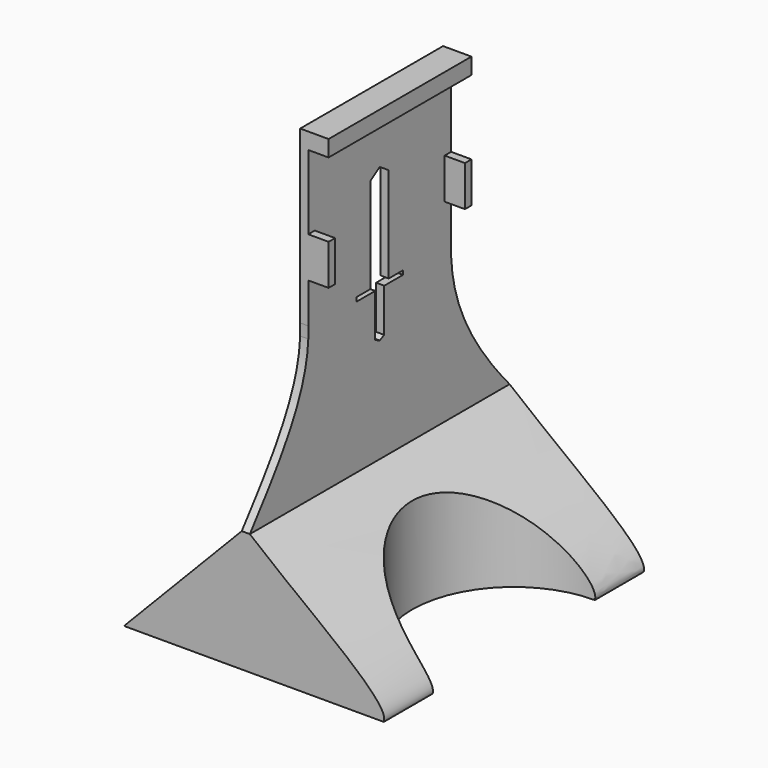
from build123d import *

# Parameters (mm, degrees)
F1_DEPTH  = 400
F2_R      = 75
F2_R_2    = 125
F3_DEPTH  = 160
F4_W      = 10
F4_H      = 400
F5_DEPTH  = 400
F7_DEPTH  = 369
F8_DEPTH  = 744
F9_DEPTH  = 294
F10_DEPTH = 25
F11_W     = 220
F11_H     = 20
F12_DEPTH = 25
F13_W     = 10
F13_H     = 50
F14_DEPTH = 25


with BuildPart() as f1:
    # F0 (on Front) → F1 (new body)
    with BuildSketch(Plane.XZ):
        with BuildLine():
            Line((-10, 0), (0, 0))
            Line((0, 0), (160, 0))
            add(Edge.make_bspline(
                [(160, 0), (168.8577404315, 22.9710926099), (70.8040622396, 86.9003880522), (-4.9911788106, 150)],
                knots=[0.4586039165, 0.4586039165, 0.4586039165, 0.4586039165, 1, 1, 1, 1], degree=3))
            Line((-4.9911788106, 150), (-14.9911788106, 150))
            Line((-14.9911788106, 150), (-160, 0))
            Line((-160, 0), (-60, 0))
            Line((-60, 0), (-10, 0))
        make_face()
    extrude(amount=F1_DEPTH)

    # F2 (on face) → F3 (cut)
    with BuildSketch(Plane(origin=(0, 0, 0), x_dir=(1, 0, 0), z_dir=(0, 0, -1))):
        with Locations((-160, 200)):
            Circle(F2_R)
        with Locations((160, 200)):
            Circle(F2_R_2)
    extrude(amount=-F3_DEPTH, mode=Mode.SUBTRACT)

    # F4 (on face) → F5 (join)
    with BuildSketch(Plane.XY.offset(150)):
        with Locations((-9.9911788106, -200)):
            Rectangle(F4_W, F4_H)
    extrude(amount=F5_DEPTH)

    # F6 (on face) → F7 (cut)
    with BuildSketch(Plane.YZ.offset(-4.9911788106)):
        with BuildLine():
            Line((-400, 550), (-400, 150))
            add(Edge.make_bspline(
                [(-400, 150), (-356.3451728041, 206.1467944777), (-312.9584078924, 262.3039541318), (-310, 325.0278234482)],
                knots=[0, 0, 0, 0, 0.4740286783, 0.4740286783, 0.4740286783, 0.4740286783], degree=3))
            Line((-310, 325.0278234482), (-310, 339.2202581751))
            add(Edge.make_bspline(
                [(-310, 339.2202581751), (-312.9911644459, 405.1052836748), (-356.3650932552, 477.5474537124), (-400, 550)],
                knots=[0.5095094707, 0.5095094707, 0.5095094707, 0.5095094707, 1, 1, 1, 1], degree=3))
        make_face()
        with BuildLine():
            Line((0, 550), (-90, 550))
            Line((-90, 550), (-90, 530))
            Line((-90, 530), (-90, 340.4403127563))
            add(Edge.make_bspline(
                [(0, 550), (-49.5785227153, 477.7428221558), (-87.2010209493, 405.969304948), (-90, 340.4403127563)],
                knots=[0, 0, 0, 0, 0.4874574601, 0.4874574601, 0.4874574601, 0.4874574601], degree=3))
        make_face()
        with BuildLine():
            Line((-310, 339.2202581751), (-310, 325.0278234482))
            add(Edge.make_bspline(
                [(-310, 325.0278234482), (-309.7785647553, 329.7226714383), (-309.7836270458, 334.4543090401), (-310, 339.2202581751)],
                knots=[0.4740286783, 0.4740286783, 0.4740286783, 0.4740286783, 0.5095094707, 0.5095094707, 0.5095094707, 0.5095094707], degree=3))
        make_face()
        with BuildLine():
            Line((-310, 550), (-400, 550))
            add(Edge.make_bspline(
                [(-310, 339.2202581751), (-312.9911644459, 405.1052836748), (-356.3650932552, 477.5474537124), (-400, 550)],
                knots=[0.5095094707, 0.5095094707, 0.5095094707, 0.5095094707, 1, 1, 1, 1], degree=3))
            Line((-310, 339.2202581751), (-310, 530))
            Line((-310, 530), (-310, 550))
        make_face()
        with BuildLine():
            Line((0, 150), (0, 550))
            add(Edge.make_bspline(
                [(0, 550), (-49.5785227153, 477.7428221558), (-87.2010209493, 405.969304948), (-90, 340.4403127563)],
                knots=[0, 0, 0, 0, 0.4874574601, 0.4874574601, 0.4874574601, 0.4874574601], degree=3))
            Line((-90, 340.4403127563), (-90, 325.0278234482))
            add(Edge.make_bspline(
                [(-90, 325.0278234482), (-87.2318561535, 262.2986085933), (-49.8238669759, 205.9050330021), (0, 150)],
                knots=[0.5259713217, 0.5259713217, 0.5259713217, 0.5259713217, 1, 1, 1, 1], degree=3))
        make_face()
        with BuildLine():
            Line((-90, 325.0278234482), (-90, 340.4403127563))
            add(Edge.make_bspline(
                [(-90, 340.4403127563), (-90.2211464603, 335.2628875556), (-90.224906032, 330.1244439943), (-90, 325.0278234482)],
                knots=[0.4874574601, 0.4874574601, 0.4874574601, 0.4874574601, 0.5259713217, 0.5259713217, 0.5259713217, 0.5259713217], degree=3))
        make_face()
        Polygon((-186.1447365284, 340.2760970592), (-186.1447365284, 457.7941475637), (-200, 466.9407904148), (-213.8552634716, 457.7941475637), (-213.8552634716, 340.2760970592), (-225.8552634716, 340.2760970592), (-235.8552634716, 340.2760970592), (-235.8552634716, 335.2760970592), (-213.8552634716, 335.2760970592), (-206.9276317358, 335.2760970592), (-206.9276317358, 281.9714009762), (-200, 278.6667048931), (-193.0723682642, 281.9714009762), (-193.0723682642, 335.2760970592), (-186.1447365284, 335.2760970592), (-164.1447365284, 335.2760970592), (-164.1447365284, 340.2760970592), (-174.1447365284, 340.2760970592), align=None)
    extrude(amount=-F7_DEPTH, mode=Mode.SUBTRACT)

    # F6 (on face) → F8 (cut)
    with BuildSketch(Plane.YZ.offset(-4.9911788106)):
        with BuildLine():
            Line((-400, 550), (-400, 150))
            add(Edge.make_bspline(
                [(-400, 150), (-356.3451728041, 206.1467944777), (-312.9584078924, 262.3039541318), (-310, 325.0278234482)],
                knots=[0, 0, 0, 0, 0.4740286783, 0.4740286783, 0.4740286783, 0.4740286783], degree=3))
            Line((-310, 325.0278234482), (-310, 339.2202581751))
            add(Edge.make_bspline(
                [(-310, 339.2202581751), (-312.9911644459, 405.1052836748), (-356.3650932552, 477.5474537124), (-400, 550)],
                knots=[0.5095094707, 0.5095094707, 0.5095094707, 0.5095094707, 1, 1, 1, 1], degree=3))
        make_face()
        with BuildLine():
            Line((0, 550), (-90, 550))
            Line((-90, 550), (-90, 530))
            Line((-90, 530), (-90, 340.4403127563))
            add(Edge.make_bspline(
                [(0, 550), (-49.5785227153, 477.7428221558), (-87.2010209493, 405.969304948), (-90, 340.4403127563)],
                knots=[0, 0, 0, 0, 0.4874574601, 0.4874574601, 0.4874574601, 0.4874574601], degree=3))
        make_face()
        with BuildLine():
            Line((-310, 339.2202581751), (-310, 325.0278234482))
            add(Edge.make_bspline(
                [(-310, 325.0278234482), (-309.7785647553, 329.7226714383), (-309.7836270458, 334.4543090401), (-310, 339.2202581751)],
                knots=[0.4740286783, 0.4740286783, 0.4740286783, 0.4740286783, 0.5095094707, 0.5095094707, 0.5095094707, 0.5095094707], degree=3))
        make_face()
        with BuildLine():
            Line((-310, 550), (-400, 550))
            add(Edge.make_bspline(
                [(-310, 339.2202581751), (-312.9911644459, 405.1052836748), (-356.3650932552, 477.5474537124), (-400, 550)],
                knots=[0.5095094707, 0.5095094707, 0.5095094707, 0.5095094707, 1, 1, 1, 1], degree=3))
            Line((-310, 339.2202581751), (-310, 530))
            Line((-310, 530), (-310, 550))
        make_face()
        with BuildLine():
            Line((0, 150), (0, 550))
            add(Edge.make_bspline(
                [(0, 550), (-49.5785227153, 477.7428221558), (-87.2010209493, 405.969304948), (-90, 340.4403127563)],
                knots=[0, 0, 0, 0, 0.4874574601, 0.4874574601, 0.4874574601, 0.4874574601], degree=3))
            Line((-90, 340.4403127563), (-90, 325.0278234482))
            add(Edge.make_bspline(
                [(-90, 325.0278234482), (-87.2318561535, 262.2986085933), (-49.8238669759, 205.9050330021), (0, 150)],
                knots=[0.5259713217, 0.5259713217, 0.5259713217, 0.5259713217, 1, 1, 1, 1], degree=3))
        make_face()
        with BuildLine():
            Line((-90, 325.0278234482), (-90, 340.4403127563))
            add(Edge.make_bspline(
                [(-90, 340.4403127563), (-90.2211464603, 335.2628875556), (-90.224906032, 330.1244439943), (-90, 325.0278234482)],
                knots=[0.4874574601, 0.4874574601, 0.4874574601, 0.4874574601, 0.5259713217, 0.5259713217, 0.5259713217, 0.5259713217], degree=3))
        make_face()
        Polygon((-186.1447365284, 340.2760970592), (-186.1447365284, 457.7941475637), (-200, 466.9407904148), (-213.8552634716, 457.7941475637), (-213.8552634716, 340.2760970592), (-225.8552634716, 340.2760970592), (-235.8552634716, 340.2760970592), (-235.8552634716, 335.2760970592), (-213.8552634716, 335.2760970592), (-206.9276317358, 335.2760970592), (-206.9276317358, 281.9714009762), (-200, 278.6667048931), (-193.0723682642, 281.9714009762), (-193.0723682642, 335.2760970592), (-186.1447365284, 335.2760970592), (-164.1447365284, 335.2760970592), (-164.1447365284, 340.2760970592), (-174.1447365284, 340.2760970592), align=None)
    extrude(amount=-F8_DEPTH, mode=Mode.SUBTRACT)

    # F6 (on face) → F9 (cut)
    with BuildSketch(Plane.YZ.offset(-4.9911788106)):
        with BuildLine():
            Line((-400, 550), (-400, 150))
            add(Edge.make_bspline(
                [(-400, 150), (-356.3451728041, 206.1467944777), (-312.9584078924, 262.3039541318), (-310, 325.0278234482)],
                knots=[0, 0, 0, 0, 0.4740286783, 0.4740286783, 0.4740286783, 0.4740286783], degree=3))
            Line((-310, 325.0278234482), (-310, 339.2202581751))
            add(Edge.make_bspline(
                [(-310, 339.2202581751), (-312.9911644459, 405.1052836748), (-356.3650932552, 477.5474537124), (-400, 550)],
                knots=[0.5095094707, 0.5095094707, 0.5095094707, 0.5095094707, 1, 1, 1, 1], degree=3))
        make_face()
        with BuildLine():
            Line((0, 550), (-90, 550))
            Line((-90, 550), (-90, 530))
            Line((-90, 530), (-90, 340.4403127563))
            add(Edge.make_bspline(
                [(0, 550), (-49.5785227153, 477.7428221558), (-87.2010209493, 405.969304948), (-90, 340.4403127563)],
                knots=[0, 0, 0, 0, 0.4874574601, 0.4874574601, 0.4874574601, 0.4874574601], degree=3))
        make_face()
        with BuildLine():
            Line((-310, 339.2202581751), (-310, 325.0278234482))
            add(Edge.make_bspline(
                [(-310, 325.0278234482), (-309.7785647553, 329.7226714383), (-309.7836270458, 334.4543090401), (-310, 339.2202581751)],
                knots=[0.4740286783, 0.4740286783, 0.4740286783, 0.4740286783, 0.5095094707, 0.5095094707, 0.5095094707, 0.5095094707], degree=3))
        make_face()
        with BuildLine():
            Line((-310, 550), (-400, 550))
            add(Edge.make_bspline(
                [(-310, 339.2202581751), (-312.9911644459, 405.1052836748), (-356.3650932552, 477.5474537124), (-400, 550)],
                knots=[0.5095094707, 0.5095094707, 0.5095094707, 0.5095094707, 1, 1, 1, 1], degree=3))
            Line((-310, 339.2202581751), (-310, 530))
            Line((-310, 530), (-310, 550))
        make_face()
        with BuildLine():
            Line((0, 150), (0, 550))
            add(Edge.make_bspline(
                [(0, 550), (-49.5785227153, 477.7428221558), (-87.2010209493, 405.969304948), (-90, 340.4403127563)],
                knots=[0, 0, 0, 0, 0.4874574601, 0.4874574601, 0.4874574601, 0.4874574601], degree=3))
            Line((-90, 340.4403127563), (-90, 325.0278234482))
            add(Edge.make_bspline(
                [(-90, 325.0278234482), (-87.2318561535, 262.2986085933), (-49.8238669759, 205.9050330021), (0, 150)],
                knots=[0.5259713217, 0.5259713217, 0.5259713217, 0.5259713217, 1, 1, 1, 1], degree=3))
        make_face()
        with BuildLine():
            Line((-90, 325.0278234482), (-90, 340.4403127563))
            add(Edge.make_bspline(
                [(-90, 340.4403127563), (-90.2211464603, 335.2628875556), (-90.224906032, 330.1244439943), (-90, 325.0278234482)],
                knots=[0.4874574601, 0.4874574601, 0.4874574601, 0.4874574601, 0.5259713217, 0.5259713217, 0.5259713217, 0.5259713217], degree=3))
        make_face()
        Polygon((-186.1447365284, 340.2760970592), (-186.1447365284, 457.7941475637), (-200, 466.9407904148), (-213.8552634716, 457.7941475637), (-213.8552634716, 340.2760970592), (-225.8552634716, 340.2760970592), (-235.8552634716, 340.2760970592), (-235.8552634716, 335.2760970592), (-213.8552634716, 335.2760970592), (-206.9276317358, 335.2760970592), (-206.9276317358, 281.9714009762), (-200, 278.6667048931), (-193.0723682642, 281.9714009762), (-193.0723682642, 335.2760970592), (-186.1447365284, 335.2760970592), (-164.1447365284, 335.2760970592), (-164.1447365284, 340.2760970592), (-174.1447365284, 340.2760970592), align=None)
    extrude(amount=-F9_DEPTH, mode=Mode.SUBTRACT)

    # F6 (on face) → F10 (cut)
    with BuildSketch(Plane.YZ.offset(-4.9911788106)):
        with BuildLine():
            Line((-400, 550), (-400, 150))
            add(Edge.make_bspline(
                [(-400, 150), (-356.3451728041, 206.1467944777), (-312.9584078924, 262.3039541318), (-310, 325.0278234482)],
                knots=[0, 0, 0, 0, 0.4740286783, 0.4740286783, 0.4740286783, 0.4740286783], degree=3))
            Line((-310, 325.0278234482), (-310, 339.2202581751))
            add(Edge.make_bspline(
                [(-310, 339.2202581751), (-312.9911644459, 405.1052836748), (-356.3650932552, 477.5474537124), (-400, 550)],
                knots=[0.5095094707, 0.5095094707, 0.5095094707, 0.5095094707, 1, 1, 1, 1], degree=3))
        make_face()
        with BuildLine():
            Line((0, 550), (-90, 550))
            Line((-90, 550), (-90, 530))
            Line((-90, 530), (-90, 340.4403127563))
            add(Edge.make_bspline(
                [(0, 550), (-49.5785227153, 477.7428221558), (-87.2010209493, 405.969304948), (-90, 340.4403127563)],
                knots=[0, 0, 0, 0, 0.4874574601, 0.4874574601, 0.4874574601, 0.4874574601], degree=3))
        make_face()
        with BuildLine():
            Line((-310, 339.2202581751), (-310, 325.0278234482))
            add(Edge.make_bspline(
                [(-310, 325.0278234482), (-309.7785647553, 329.7226714383), (-309.7836270458, 334.4543090401), (-310, 339.2202581751)],
                knots=[0.4740286783, 0.4740286783, 0.4740286783, 0.4740286783, 0.5095094707, 0.5095094707, 0.5095094707, 0.5095094707], degree=3))
        make_face()
        with BuildLine():
            Line((-310, 550), (-400, 550))
            add(Edge.make_bspline(
                [(-310, 339.2202581751), (-312.9911644459, 405.1052836748), (-356.3650932552, 477.5474537124), (-400, 550)],
                knots=[0.5095094707, 0.5095094707, 0.5095094707, 0.5095094707, 1, 1, 1, 1], degree=3))
            Line((-310, 339.2202581751), (-310, 530))
            Line((-310, 530), (-310, 550))
        make_face()
        with BuildLine():
            Line((0, 150), (0, 550))
            add(Edge.make_bspline(
                [(0, 550), (-49.5785227153, 477.7428221558), (-87.2010209493, 405.969304948), (-90, 340.4403127563)],
                knots=[0, 0, 0, 0, 0.4874574601, 0.4874574601, 0.4874574601, 0.4874574601], degree=3))
            Line((-90, 340.4403127563), (-90, 325.0278234482))
            add(Edge.make_bspline(
                [(-90, 325.0278234482), (-87.2318561535, 262.2986085933), (-49.8238669759, 205.9050330021), (0, 150)],
                knots=[0.5259713217, 0.5259713217, 0.5259713217, 0.5259713217, 1, 1, 1, 1], degree=3))
        make_face()
        with BuildLine():
            Line((-90, 325.0278234482), (-90, 340.4403127563))
            add(Edge.make_bspline(
                [(-90, 340.4403127563), (-90.2211464603, 335.2628875556), (-90.224906032, 330.1244439943), (-90, 325.0278234482)],
                knots=[0.4874574601, 0.4874574601, 0.4874574601, 0.4874574601, 0.5259713217, 0.5259713217, 0.5259713217, 0.5259713217], degree=3))
        make_face()
        Polygon((-186.1447365284, 340.2760970592), (-186.1447365284, 457.7941475637), (-200, 466.9407904148), (-213.8552634716, 457.7941475637), (-213.8552634716, 340.2760970592), (-225.8552634716, 340.2760970592), (-235.8552634716, 340.2760970592), (-235.8552634716, 335.2760970592), (-213.8552634716, 335.2760970592), (-206.9276317358, 335.2760970592), (-206.9276317358, 281.9714009762), (-200, 278.6667048931), (-193.0723682642, 281.9714009762), (-193.0723682642, 335.2760970592), (-186.1447365284, 335.2760970592), (-164.1447365284, 335.2760970592), (-164.1447365284, 340.2760970592), (-174.1447365284, 340.2760970592), align=None)
    extrude(amount=-F10_DEPTH, mode=Mode.SUBTRACT)

    # F11 (on face) → F12 (join)
    with BuildSketch(Plane.YZ.offset(-4.9911788106)):
        with Locations((-200, 540)):
            Rectangle(F11_W, F11_H)
    extrude(amount=F12_DEPTH)

    # F13 (on face) → F14 (join)
    with BuildSketch(Plane.YZ.offset(-4.9911788106)):
        with Locations((-305, 413.565659523)):
            Rectangle(F13_W, F13_H)
        with Locations((-95, 413.565659523)):
            Rectangle(F13_W, F13_H)
    extrude(amount=F14_DEPTH)


solid = f1.part
